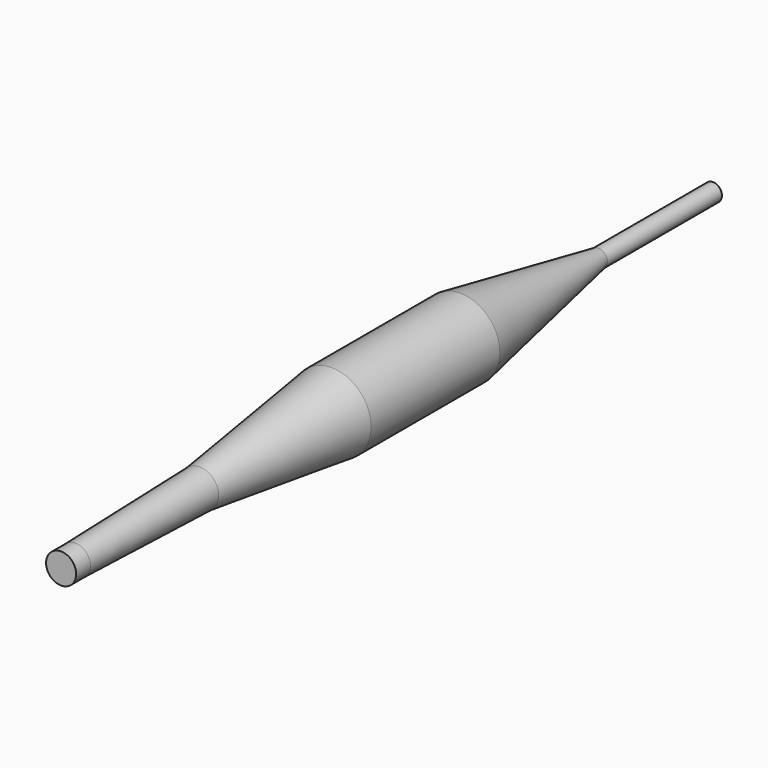
from build123d import *

# Parameters (mm, degrees)
F0_W   = 25
F0_H   = 21
F0_W_2 = 224.9109574539
F0_H_2 = 55
F0_W_3 = 200
F0_H_3 = 12.5


# Not quite as in the source:
# - the program builds the solid bodies; features that only make, move or delete a surface that nothing else refers to are left out


with BuildPart() as f1:
    # F0 (on Right) → F1 (revolve)
    with BuildSketch(Plane.YZ):
        with Locations((12.5, 223.4762815751)):
            Rectangle(F0_W, F0_H)
        Polygon((25, 233.9762815751), (25, 212.9762815751), (242, 212.9762815751), (242, 239.6586265556), align=None)
        Polygon((242, 239.6586265556), (242, 212.9762815751), (344.0616714118, 212.9762815751), (344.0616714118, 252.1902240649), align=None)
        Polygon((344.0616714118, 252.1902240649), (344.0616714118, 212.9762815751), (472.6287925066, 212.9762815751), (472.6287925066, 267.9762815751), align=None)
        with Locations((585.0842712335, 240.4762815751)):
            Rectangle(F0_W_2, F0_H_2)
        Polygon((697.5397499605, 267.9762815751), (697.5397499605, 212.9762815751), (853.5, 212.9762815751), (853.5, 240.4762815751), align=None)
        Polygon((853.5, 240.4762815751), (853.5, 212.9762815751), (938.5692272943, 212.9762815751), (938.5692272943, 225.4762815751), align=None)
        with Locations((1038.5692272943, 219.2262815751)):
            Rectangle(F0_W_3, F0_H_3)
    revolve(axis=Axis((0, -32.5, 212.9762815751), (0, -1, 0)))


solid = f1.part
